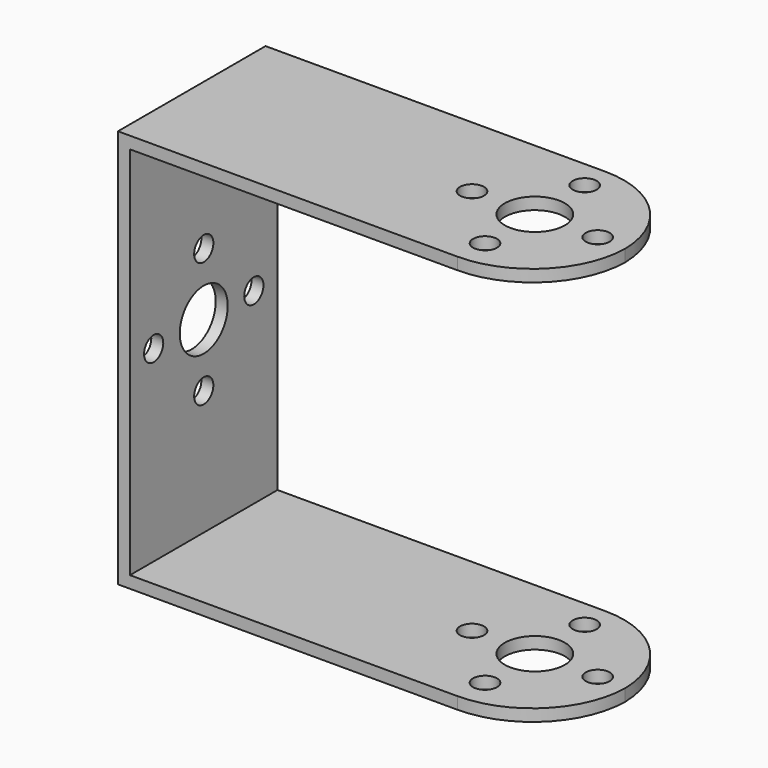
from build123d import *

# Parameters (mm, degrees)
F1_DEPTH    = 24.6
F2_T1_DEPTH = 64.1
F3_T1_DEPTH = 64.1
F4_R        = 4
F4_R_2      = 1.6
F5_DEPTH    = 100
F6_R        = 4
F6_R_2      = 1.6
F7_DEPTH    = 1.6


# Not quite as in the source:
# - a fillet or chamfer that OpenCascade refuses, or shapes differently, is made with other operations: its cross-section is extruded or revolved along the edge and cut away or added


with BuildPart() as f1:
    # F0 (on Front) → F1 (new body)
    with BuildSketch(Plane.XZ):
        Polygon((-28.9, -26.6), (28.9, -26.6), (28.9, -25), (-27.3, -25), (-27.3, 25), (28.9, 25), (28.9, 26.6), (-28.9, 26.6), align=None)
    extrude(amount=F1_DEPTH)

    # F2: fillet of radius 12.5 on 2 edges, made by hand

    # F2_s2 → F2_t1 (cut)
    with BuildSketch(Plane.XY.offset(-57.85)):
        with BuildLine():
            ThreePointArc((28.9, -12.1), (25.2388347648, -20.9388347648), (16.4, -24.6))
            Line((16.4, -24.6), (28.9, -24.6))
            Line((28.9, -24.6), (28.9, -12.1))
        make_face()
        with BuildLine():
            ThreePointArc((28.9, -12.5), (25.2388347648, -3.6611652352), (16.4, 0))
            Line((16.4, 0), (28.9, 0))
            Line((28.9, 0), (28.9, -12.5))
        make_face()
    extrude(amount=F2_T1_DEPTH, mode=Mode.SUBTRACT)

    # F3: fillet of radius 12.5 on 2 edges, made by hand

    # F3_s2 → F3_t1 (cut)
    with BuildSketch(Plane.XY.offset(-6.25)):
        with BuildLine():
            ThreePointArc((16.4, -24.6), (25.2388347648, -20.9388347648), (28.9, -12.1))
            Line((28.9, -12.1), (28.9, -24.6))
            Line((28.9, -24.6), (16.4, -24.6))
        make_face()
        with BuildLine():
            ThreePointArc((16.4, 0), (25.2388347648, -3.6611652352), (28.9, -12.5))
            Line((28.9, -12.5), (28.9, 0))
            Line((28.9, 0), (16.4, 0))
        make_face()
    extrude(amount=F3_T1_DEPTH, mode=Mode.SUBTRACT)

    # F4 (on face) → F5 (cut)
    with BuildSketch(Plane(origin=(0, 0, -26.6), x_dir=(1, 0, 0), z_dir=(0, 0, -1))):
        with Locations((16.6995614014, 12.1)):
            Circle(F4_R)
        with Locations((16.6629385944, 3.7500803136)):
            Circle(F4_R_2)
        with Locations((8.349641715, 12.136622807)):
            Circle(F4_R_2)
        with Locations((16.7361842084, 20.4499196864)):
            Circle(F4_R_2)
        with Locations((25.0494810878, 12.063377193)):
            Circle(F4_R_2)
    extrude(amount=-F5_DEPTH, mode=Mode.SUBTRACT)

    # F6 (on face) → F7 (cut)
    with BuildSketch(Plane.YZ.offset(-27.3)):
        with Locations((-12.3, 0)):
            Circle(F6_R)
        with BuildLine():
            ThreePointArc((-2.35, 0), (-3.95, 1.6), (-5.55, 0))
            ThreePointArc((-5.55, 0), (-3.95, -1.6), (-2.35, 0))
        make_face()
        with Locations((-12.3, 8.35)):
            Circle(F6_R_2)
        with Locations((-20.65, 0)):
            Circle(F6_R_2)
        with Locations((-12.3, -8.35)):
            Circle(F6_R_2)
    extrude(amount=-F7_DEPTH, mode=Mode.SUBTRACT)


solid = f1.part
